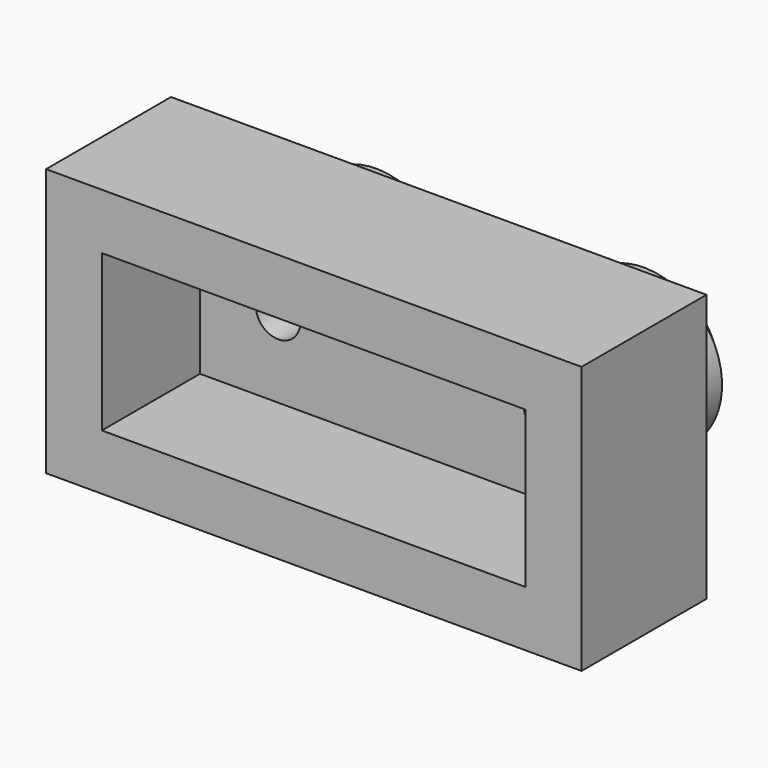
from build123d import *

# Parameters (mm, degrees)
F0_W     = 76.2
F0_H     = 38.1
F1_DEPTH = 25.4
F2_R     = 11.1125
F3_DEPTH = 12.7
F4_SIZE2 = 3.175
F4_SIZE  = 3.175
F5_T     = 7.9375


# Not quite as in the source:
# - a shell that OpenCascade refuses in one call is made with other operations: the cavity is built on its own and cut out


with BuildPart() as f1:
    # F0 (on Front) → F1 (new body)
    with BuildSketch(Plane.XZ):
        Rectangle(F0_W, F0_H)
    extrude(amount=F1_DEPTH)

    # F2 (on face) → F3 (join)
    with BuildSketch(Plane(origin=(0, 0, 0), x_dir=(-1, 0, 0), z_dir=(0, 1, 0))):
        with Locations((-19.05, 0)):
            Circle(F2_R)
        with Locations((19.05, 0)):
            Circle(F2_R)
    extrude(amount=F3_DEPTH)

    # F4
    f4_edges = [f1.edges().sort_by_distance(p)[0] for p in [
        (-7.9375, 12.7, 0),
        (30.1625, 12.7, 0),
        (0, 0, 19.05),
        (38.1, 0, 0),
        (-38.1, 0, 0),
        (0, 0, -19.05),
    ]]
    chamfer(f4_edges, length=F4_SIZE, length2=F4_SIZE2)

    # F5: shell of thickness 7.9375, made by hand


with BuildPart() as f5_core1:
    # F5_t2: copy of F1
    add(f1.part)

    # the walls: a layer under each face that stays
    f5_faces = [f5_core1.faces().sort_by_distance(p)[0] for p in [
        (0, -14.2875, -19.05),
        (-38.1, -14.2875, 0),
        (0, -1.5875, -17.4625),
        (38.1, -14.2875, 0),
        (0, -14.2875, 19.05),
        (-36.5125, -1.5875, 0),
        (0, 0, 0),
        (36.5125, -1.5875, 0),
        (0, -1.5875, 17.4625),
        (-7.9375, 4.7625, 0),
        (30.1625, 4.7625, 0),
        (-9.525, 11.1125, 0),
        (28.575, 11.1125, 0),
        (-19.05, 12.7, 0),
        (19.05, 12.7, 0),
    ]]
    thicken(f5_faces, amount=-F5_T, mode=Mode.SUBTRACT)

    # F5_s3 → F5_t4 (revolve, cut)
    with BuildSketch(Plane.XY):
        Polygon((-30.241875, 0.079375), (-30.1625, -7.9375), (-22.225, -7.9375), (-22.225, 0), align=None)
    revolve(axis=Axis((-19.05, 0, 0), (0, 1, 0)), mode=Mode.SUBTRACT)

    # F5_s5 → F5_t6 (revolve, cut)
    with BuildSketch(Plane.XY):
        Polygon((7.858125, 0.079375), (7.9375, -7.9375), (15.875, -7.9375), (15.875, 0), align=None)
    revolve(axis=Axis((19.05, 0, 0), (0, 1, 0)), mode=Mode.SUBTRACT)


with BuildPart() as f1_1:
    add(f1.part)

    # what is left inside the walls is the cavity
    f5_cavity = [f5_core1.part.solids().sort_by_distance(p)[0] for p in [
        (0, -25.320625, -3.704167),
    ]]
    add(f5_cavity, mode=Mode.SUBTRACT)


solid = f1_1.part
